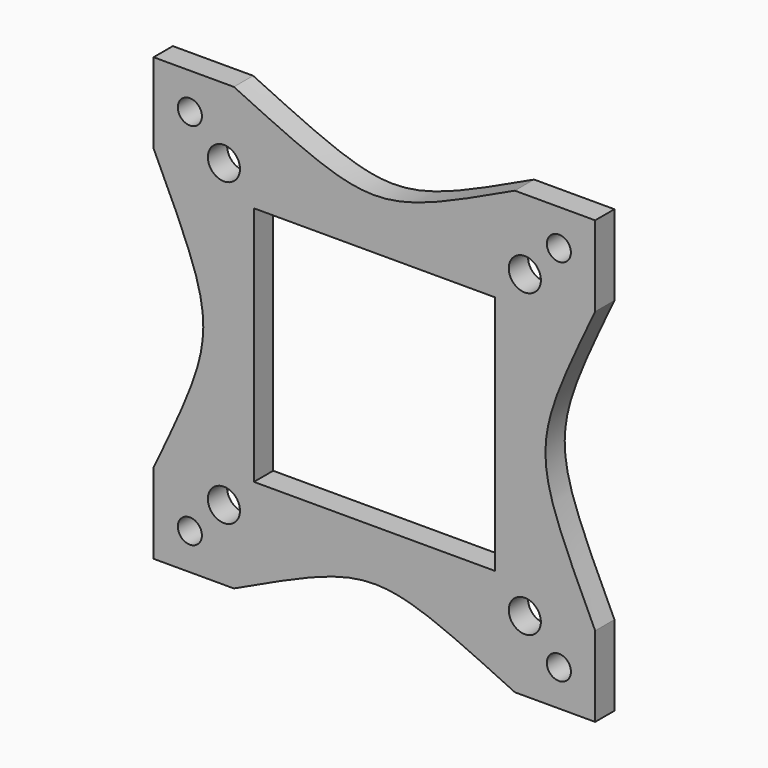
from build123d import *

# Parameters (mm, degrees)
F0_R     = 1.5
F0_R_2   = 2
F0_W     = 30
F0_H     = 30
F1_DEPTH = 3


# Not quite as in the source:
# - ends of sketch curves that miss each other by under 0.0002 mm in the source are joined


with BuildPart() as f1:
    # F0 (on Front) → F1 (new body)
    with BuildSketch(Plane.XZ):
        with BuildLine():
            Line((27.5, 17.5), (27.5, 27.5))
            Line((27.5, 27.5), (17.5, 27.5))
            add(Edge.make_bspline(
                [(17.5, 27.5), (0, 19.2440692335), (0, 19.2440692335), (-17.5, 27.5)],
                knots=[0, 0, 0, 0, 35, 35, 35, 35], degree=3))
            Line((-17.5, 27.5), (-27.5, 27.5))
            Line((-27.5, 27.5), (-27.5, 17.5))
            add(Edge.make_bspline(
                [(-27.5, 17.5), (-19.2440692335, 0), (-19.2440692335, 0), (-27.5, -17.5)],
                knots=[0, 0, 0, 0, 35, 35, 35, 35], degree=3))
            Line((-27.5, -17.5), (-27.5, -27.5))
            Line((-27.5, -27.5), (-17.5, -27.5))
            add(Edge.make_bspline(
                [(-17.5, -27.5), (0, -19.2440692335), (0, -19.2440692335), (17.5, -27.5)],
                knots=[0, 0, 0, 0, 35, 35, 35, 35], degree=3))
            Line((17.5, -27.5), (27.5, -27.5))
            Line((27.5, -27.5), (27.5, -17.5))
            add(Edge.make_bspline(
                [(27.5, -17.5), (19.2440690845, 0), (19.2440692335, 0), (27.5, 17.5)],
                knots=[0, 0, 0, 0, 35, 35, 35, 35], degree=3))
        make_face()
        with Locations((-22.9809703886, -22.9809703886)):
            Circle(F0_R, mode=Mode.SUBTRACT)
        with Locations((-18.7383297014, -18.7383297014)):
            Circle(F0_R_2, mode=Mode.SUBTRACT)
        with Locations((22.9809703886, -22.9809703886)):
            Circle(F0_R, mode=Mode.SUBTRACT)
        with Locations((18.7383297014, -18.7383297014)):
            Circle(F0_R_2, mode=Mode.SUBTRACT)
        with Locations((-18.7383297014, 18.7383297014)):
            Circle(F0_R_2, mode=Mode.SUBTRACT)
        with Locations((-22.9809703886, 22.9809703886)):
            Circle(F0_R, mode=Mode.SUBTRACT)
        Rectangle(F0_W, F0_H, mode=Mode.SUBTRACT)
        with Locations((18.7383297014, 18.7383297014)):
            Circle(F0_R_2, mode=Mode.SUBTRACT)
        with Locations((22.9809703886, 22.9809703886)):
            Circle(F0_R, mode=Mode.SUBTRACT)
    extrude(amount=F1_DEPTH)


solid = f1.part
